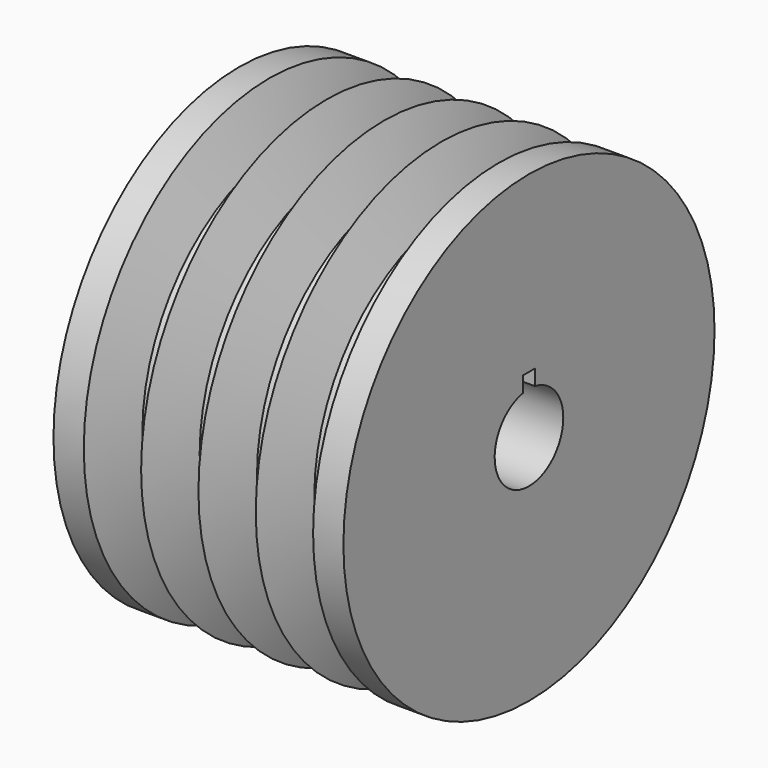
from build123d import *

# Parameters (mm, degrees)
F2_R     = 11.5
F3_DEPTH = 80.518
F5_DEPTH = 40


# Not quite as in the source:
# - ends of sketch curves that miss each other by under 0.0002 mm in the source are joined


with BuildPart() as f1:
    # F0 (on Front) → F1 (revolve)
    with BuildSketch(Plane.XZ):
        Polygon((-30.76, 31.115), (-38.89375, 31.115), (-38.89375, -31.115), (-30.76, -31.115), (30.76, -31.115), (38.89375, -31.115), (38.89375, 31.115), (30.76, 31.115), (25.8486765474, 17.62125), (20.2913232706, 17.62125), (15.379999922, 31.115), (10.4686765734, 17.62125), (4.9113232966, 17.62125), (-5.2e-08, 31.115), (-4.9113234006, 17.62125), (-10.4686766774, 17.62125), (-15.380000026, 31.115), (-20.2913233746, 17.62125), (-25.8486766514, 17.62125), align=None)
    revolve(axis=Axis((0, 0, -31.115), (1, 0, 0)))

    # F2 (on face) → F3 (cut)
    with BuildSketch(Plane.YZ.offset(38.89375)):
        with Locations((0, -31.115)):
            Circle(F2_R)
    extrude(amount=-F3_DEPTH, mode=Mode.SUBTRACT)

    # F4 (on face) → F5 (cut)
    with BuildSketch(Plane.YZ.offset(38.89375)):
        with BuildLine():
            Line((2, -15.615), (0, -15.615))
            Line((0, -15.615), (-2, -15.615))
            Line((-2, -15.615), (-2, -19.7902483471))
            ThreePointArc((-2, -19.7902483471), (0, -19.615), (2, -19.7902483471))
            Line((2, -19.7902483471), (2, -15.615))
        make_face()
    extrude(amount=-F5_DEPTH, mode=Mode.SUBTRACT)


solid = f1.part
